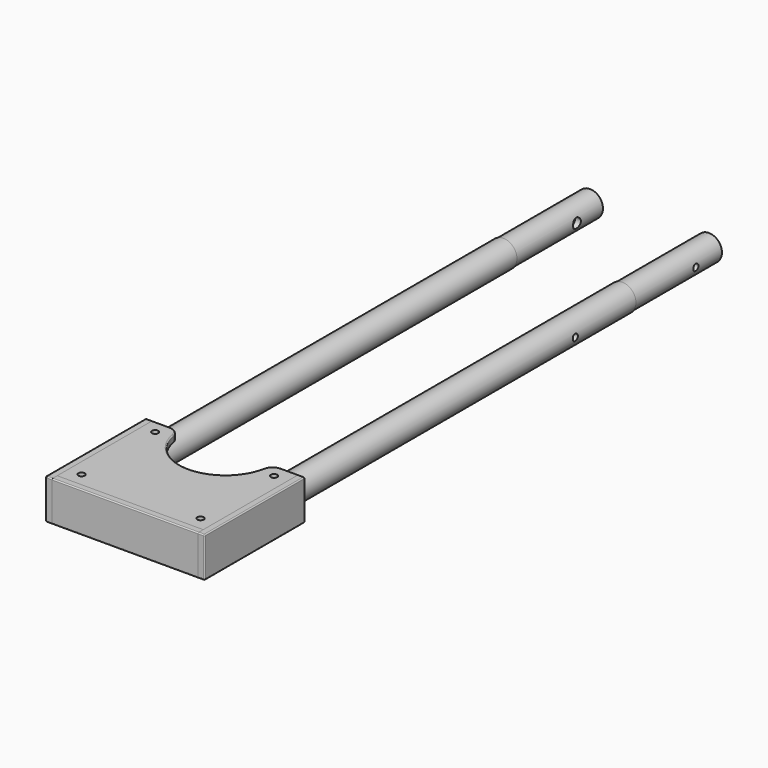
from build123d import *

# Parameters (mm, degrees)
F0_R      = 12.5
F0_R_2    = 12
F1_DEPTH  = 500
F3_R      = 3
F4_DEPTH  = 5
F8_DEPTH  = 6
F9_R      = 10
F10_R     = 3
F11_DEPTH = 31.0010001
F13_R     = 12
F14_DEPTH = 100
F16_R     = 3
F17_DEPTH = 25.0010001
F18_R     = 4.5
F19_DEPTH = 6
F21_R     = 4.75
F22_DEPTH = 6
F23_W     = 135
F23_H     = 37
F24_DEPTH = 6
F25_W     = 116
F25_H     = 37
F26_DEPTH = 6
F28_R     = 1
F28_2_R   = 1
F28_3_R   = 1
F28_4_R   = 1
F28_5_R   = 1


# Not quite as in the source:
# - a feature names something its author has since deleted; it is built from what else it names


with BuildPart() as f1:
    # F0 (on Front) → F1 (new body)
    with BuildSketch(Plane.XZ):
        with Locations((-55, 0)):
            Circle(F0_R)
        with Locations((-55, 0)):
            Circle(F0_R_2, mode=Mode.SUBTRACT)
    extrude(amount=-F1_DEPTH)

    # F3 (on offset) → F4 (cut)
    with BuildSketch(Plane.YZ.offset(-67.5)):
        with Locations((430, 0)):
            Circle(F3_R)
    extrude(amount=F4_DEPTH, mode=Mode.SUBTRACT)


with BuildPart() as f5_1:
    # F5: instance of F1
    add(f1.part.mirror(Plane.YZ))


with BuildPart() as f8:
    # F7 (on offset) → F8 (new body)
    with BuildSketch(Plane.XY.offset(-12.5)):
        with BuildLine():
            Line((-42.5, 110), (-67.5, 110))
            Line((-67.5, 110), (-67.5, 0))
            Line((-67.5, 0), (67.5, 0))
            Line((67.5, 0), (67.5, 110))
            Line((67.5, 110), (42.5, 110))
            ThreePointArc((42.5, 110), (0, 67.5), (-42.5, 110))
        make_face()
    extrude(amount=-F8_DEPTH)

    # F9
    f9_edges = [f8.edges().sort_by_distance(p)[0] for p in [
        (-42.5, 110, -15.5),
        (42.5, 110, -15.5),
    ]]
    fillet(f9_edges, radius=F9_R)


with BuildPart() as f11_tool:
    # F10 (on face) → F11 (new body, through all)
    with BuildSketch(Plane(origin=(0, 0, -18.5), x_dir=(1, 0, 0), z_dir=(0, 0, -1))):
        with Locations((-55, -12.5)):
            Circle(F10_R)
        with Locations((-55, -97.5)):
            Circle(F10_R)
        with Locations((55, -97.5)):
            Circle(F10_R)
        with Locations((55, -12.5)):
            Circle(F10_R)
    extrude(amount=-F11_DEPTH)


with BuildPart() as f1_1:
    add(f1.part)

    # F11: cut by f11_tool
    add(f11_tool.part, mode=Mode.SUBTRACT)


with BuildPart() as f5_1_1:
    add(f5_1.part)

    # F11: cut by f11_tool
    add(f11_tool.part, mode=Mode.SUBTRACT)


with BuildPart() as f8_1:
    add(f8.part)

    # F11: cut by f11_tool
    add(f11_tool.part, mode=Mode.SUBTRACT)


with BuildPart() as f12_1:
    # F12: instance of F8
    add(f8_1.part.mirror(Plane.XY))

    # F28#2
    f28_2_edges = [f12_1.edges().sort_by_distance(p)[0] for p in [
        (-59.51941, 110, 18.5),
        (-45.17673, 107.715167, 18.5),
        (0, 67.5, 18.5),
        (45.17673, 107.715167, 18.5),
        (59.51941, 110, 18.5),
    ]]
    fillet(f28_2_edges, radius=F28_2_R)


with BuildPart() as f14:
    # F13 (on face) → F14 (new body, symmetric)
    with BuildSketch(Plane(origin=(0, 500, 0), x_dir=(-1, 0, 0), z_dir=(0, 1, 0))):
        with Locations((-55, 0)):
            Circle(F13_R)
    extrude(amount=F14_DEPTH, both=True)

    # F16 (on offset) → F17 (cut, through all)
    with BuildSketch(Plane.YZ.offset(42.5)):
        with Locations((430, 0)):
            Circle(F16_R)
        with Locations((570, 0)):
            Circle(F16_R)
    extrude(amount=F17_DEPTH, mode=Mode.SUBTRACT)

    # F18 (on offset) → F19 (cut)
    with BuildSketch(Plane.YZ.offset(42.5)):
        with Locations((430, 0)):
            Circle(F18_R)
        with Locations((570, 0)):
            Circle(F18_R)
    extrude(amount=F19_DEPTH, mode=Mode.SUBTRACT)


with BuildPart() as f20_1:
    # F20: instance of F14
    add(f14.part.mirror(Plane.YZ))


with BuildPart() as f8_2:
    add(f8_1.part)

    # F21 (on face) → F22 (cut, through all)
    with BuildSketch(Plane(origin=(0, 0, -18.5), x_dir=(1, 0, 0), z_dir=(0, 0, -1))):
        with Locations((0, -32)):
            Circle(F21_R)
    extrude(amount=-F22_DEPTH, mode=Mode.SUBTRACT)

    # F28
    f28_edges = [f8_2.edges().sort_by_distance(p)[0] for p in [
        (59.51941, 110, -18.5),
        (-59.51941, 110, -18.5),
        (-45.17673, 107.715167, -18.5),
        (0, 67.5, -18.5),
        (45.17673, 107.715167, -18.5),
    ]]
    fillet(f28_edges, radius=F28_R)


with BuildPart() as f24:
    # F23 (on face) → F24 (new body)
    with BuildSketch(Plane.XZ):
        Rectangle(F23_W, F23_H)
    extrude(amount=F24_DEPTH)

    # F28#3
    f28_3_edges = [f24.edges().sort_by_distance(p)[0] for p in [
        (0, -6, 18.5),
        (0, -6, -18.5),
    ]]
    fillet(f28_3_edges, radius=F28_3_R)


with BuildPart() as f26:
    # F25 (on face) → F26 (new body)
    with BuildSketch(Plane(origin=(-67.5, 0, 0), x_dir=(0, -1, 0), z_dir=(-1, 0, 0))):
        with Locations((-52, 0)):
            Rectangle(F25_W, F25_H)
    extrude(amount=F26_DEPTH)


with BuildPart() as f27_1:
    # F27: instance of F26
    add(f26.part.mirror(Plane.YZ))

    # F28#5
    f28_5_edges = [f27_1.edges().sort_by_distance(p)[0] for p in [
        (73.5, 52, 18.5),
        (70.5, -6, 18.5),
        (73.5, -6, 0),
        (73.5, 110, 0),
        (73.5, 52, -18.5),
        (70.5, -6, -18.5),
        (70.5, 110, 18.5),
        (70.5, 110, -18.5),
    ]]
    fillet(f28_5_edges, radius=F28_5_R)


with BuildPart() as f26_1:
    add(f26.part)

    # F28#4
    f28_4_edges = [f26_1.edges().sort_by_distance(p)[0] for p in [
        (-70.5, -6, -18.5),
        (-73.5, -6, 0),
        (-70.5, -6, 18.5),
        (-73.5, 52, 18.5),
        (-73.5, 52, -18.5),
        (-73.5, 110, 0),
        (-70.5, 110, 18.5),
    ]]
    fillet(f28_4_edges, radius=F28_4_R)


solid = Compound([f1_1.part, f5_1_1.part, f12_1.part, f14.part, f20_1.part, f8_2.part, f24.part, f27_1.part, f26_1.part])
